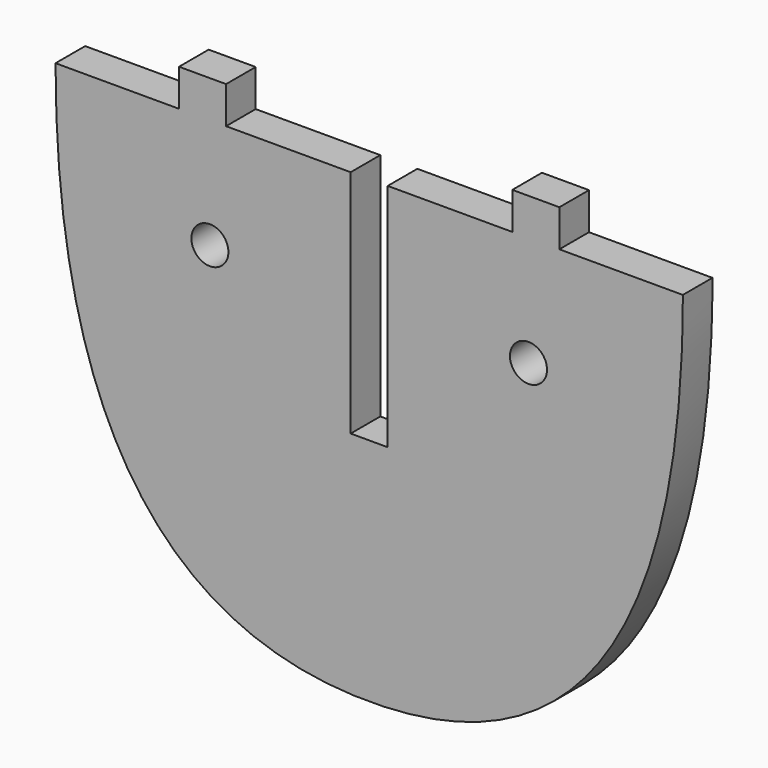
from build123d import *

# Parameters (mm, degrees)
F0_R     = 1.5
F0_W     = 3.81
F0_H     = 3
F1_DEPTH = 3


# Not quite as in the source:
# - a feature names something its author has since deleted; it is built from what else it names


with BuildPart() as f1:
    # F0 (on Front) → F1 (new body)
    with BuildSketch(Plane.XZ):
        with BuildLine():
            Line((-1.5, -18.6309), (-1.5, 0))
            Line((-1.5, 0), (-7.59, 0))
            Line((-7.59, 0), (-11.59, 0))
            Line((-11.59, 0), (-15.4, 0))
            Line((-15.4, 0), (-17.05, 0))
            Line((-17.05, 0), (-25.4, 0))
            add(Edge.make_bspline(
                [(-25.4, 0), (-25.4, -30), (-12.7, -37.25), (0, -37.25)],
                knots=[0, 0, 0, 0, 0.5, 0.5, 0.5, 0.5], degree=3))
            Line((0, -37.25), (0, -18.6309))
            Line((0, -18.6309), (-1.5, -18.6309))
        make_face()
        with Locations((-12.9, -8.9107090607)):
            Circle(F0_R, mode=Mode.SUBTRACT)
        with BuildLine():
            Line((4.35, 0), (1.5, 0))
            Line((1.5, 0), (1.5, -18.6309))
            Line((1.5, -18.6309), (0, -18.6309))
            Line((0, -18.6309), (0, -37.25))
            add(Edge.make_bspline(
                [(0, -37.25), (12.7, -37.25), (25.4, -30), (25.4, 0)],
                knots=[0.5, 0.5, 0.5, 0.5, 1, 1, 1, 1], degree=3))
            Line((25.4, 0), (15.4, 0))
            Line((15.4, 0), (11.59, 0))
            Line((11.59, 0), (6.35, 0))
            Line((6.35, 0), (4.35, 0))
        make_face()
        with Locations((12.9, -8.9107090607)):
            Circle(F0_R, mode=Mode.SUBTRACT)
        with Locations((13.495, 1.5)):
            Rectangle(F0_W, F0_H)
        with Locations((-13.495, 1.5)):
            Rectangle(F0_W, F0_H)
    extrude(amount=F1_DEPTH)


solid = f1.part
